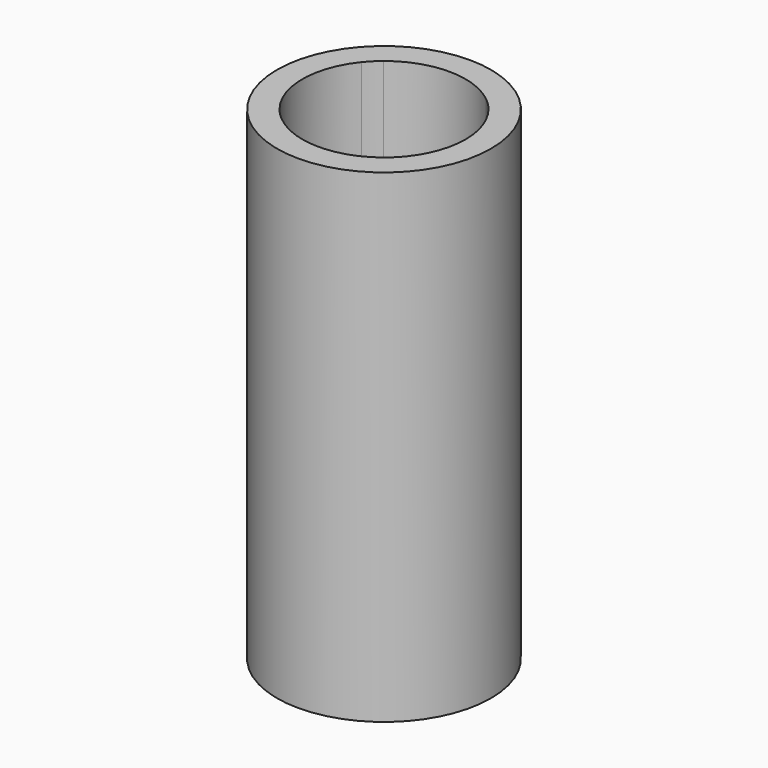
from build123d import *

# Parameters (mm, degrees)
F0_R     = 21
F0_W     = 24.95
F0_H     = 24.95
F1_DEPTH = 45
F2_R     = 21
F3_DEPTH = 50
F4_DEPTH = 5


with BuildPart() as f1:
    # F0 (on Top) → F1 (new body)
    with BuildSketch(Plane.XY):
        Circle(F0_R)
        Rectangle(F0_W, F0_H, mode=Mode.SUBTRACT)
    extrude(amount=F1_DEPTH)

    # F2 (on face) → F3 (join)
    with BuildSketch(Plane.XY.offset(45)):
        Circle(F2_R)
        with BuildLine():
            ThreePointArc((12.475, 10.0585784284), (15.1114608824, 5.3333268229), (16.025, 0))
            ThreePointArc((16.025, 0), (15.1114608824, -5.3333268229), (12.475, -10.0585784284))
            Line((12.475, -10.0585784284), (12.475, -12.475))
            Line((12.475, -12.475), (10.0585784284, -12.475))
            ThreePointArc((10.0585784284, -12.475), (0, -16.025), (-10.0585784284, -12.475))
            Line((-10.0585784284, -12.475), (-12.475, -12.475))
            Line((-12.475, -12.475), (-12.475, -10.0585784284))
            ThreePointArc((-12.475, -10.0585784284), (-16.025, 0), (-12.475, 10.0585784284))
            Line((-12.475, 10.0585784284), (-12.475, 12.475))
            Line((-12.475, 12.475), (-10.0585784284, 12.475))
            ThreePointArc((-10.0585784284, 12.475), (0, 16.025), (10.0585784284, 12.475))
            Line((10.0585784284, 12.475), (12.475, 12.475))
            Line((12.475, 12.475), (12.475, 10.0585784284))
        make_face(mode=Mode.SUBTRACT)
        with BuildLine():
            ThreePointArc((10.0585784284, 12.475), (11.3313861685, 11.3313861685), (12.475, 10.0585784284))
            Line((12.475, 10.0585784284), (12.475, 12.475))
            Line((12.475, 12.475), (10.0585784284, 12.475))
        make_face()
        with BuildLine():
            Line((12.475, -12.475), (12.475, -10.0585784284))
            ThreePointArc((12.475, -10.0585784284), (11.3313861685, -11.3313861685), (10.0585784284, -12.475))
            Line((10.0585784284, -12.475), (12.475, -12.475))
        make_face()
        with BuildLine():
            ThreePointArc((-12.475, 10.0585784284), (-11.3313861685, 11.3313861685), (-10.0585784284, 12.475))
            Line((-10.0585784284, 12.475), (-12.475, 12.475))
            Line((-12.475, 12.475), (-12.475, 10.0585784284))
        make_face()
        with BuildLine():
            Line((-12.475, -12.475), (-10.0585784284, -12.475))
            ThreePointArc((-10.0585784284, -12.475), (-11.3313861685, -11.3313861685), (-12.475, -10.0585784284))
            Line((-12.475, -10.0585784284), (-12.475, -12.475))
        make_face()
    extrude(amount=F3_DEPTH)

    # F2 (on face) → F4 (join)
    with BuildSketch(Plane.XY.offset(45)):
        with BuildLine():
            Line((12.475, -10.0585784284), (12.475, 10.0585784284))
            ThreePointArc((12.475, 10.0585784284), (11.3313861685, 11.3313861685), (10.0585784284, 12.475))
            Line((10.0585784284, 12.475), (-10.0585784284, 12.475))
            ThreePointArc((-10.0585784284, 12.475), (-11.3313861685, 11.3313861685), (-12.475, 10.0585784284))
            Line((-12.475, 10.0585784284), (-12.475, -10.0585784284))
            ThreePointArc((-12.475, -10.0585784284), (-11.3313861685, -11.3313861685), (-10.0585784284, -12.475))
            Line((-10.0585784284, -12.475), (10.0585784284, -12.475))
            ThreePointArc((10.0585784284, -12.475), (11.3313861685, -11.3313861685), (12.475, -10.0585784284))
        make_face()
        with BuildLine():
            ThreePointArc((12.475, -10.0585784284), (15.1114608824, -5.3333268229), (16.025, 0))
            ThreePointArc((16.025, 0), (15.1114608824, 5.3333268229), (12.475, 10.0585784284))
            Line((12.475, 10.0585784284), (12.475, -10.0585784284))
        make_face()
        with BuildLine():
            Line((-12.475, -10.0585784284), (-12.475, 10.0585784284))
            ThreePointArc((-12.475, 10.0585784284), (-16.025, 0), (-12.475, -10.0585784284))
        make_face()
        with BuildLine():
            ThreePointArc((-10.0585784284, -12.475), (0, -16.025), (10.0585784284, -12.475))
            Line((10.0585784284, -12.475), (-10.0585784284, -12.475))
        make_face()
        with BuildLine():
            Line((-10.0585784284, 12.475), (10.0585784284, 12.475))
            ThreePointArc((10.0585784284, 12.475), (0, 16.025), (-10.0585784284, 12.475))
        make_face()
    extrude(amount=F4_DEPTH)


solid = f1.part
